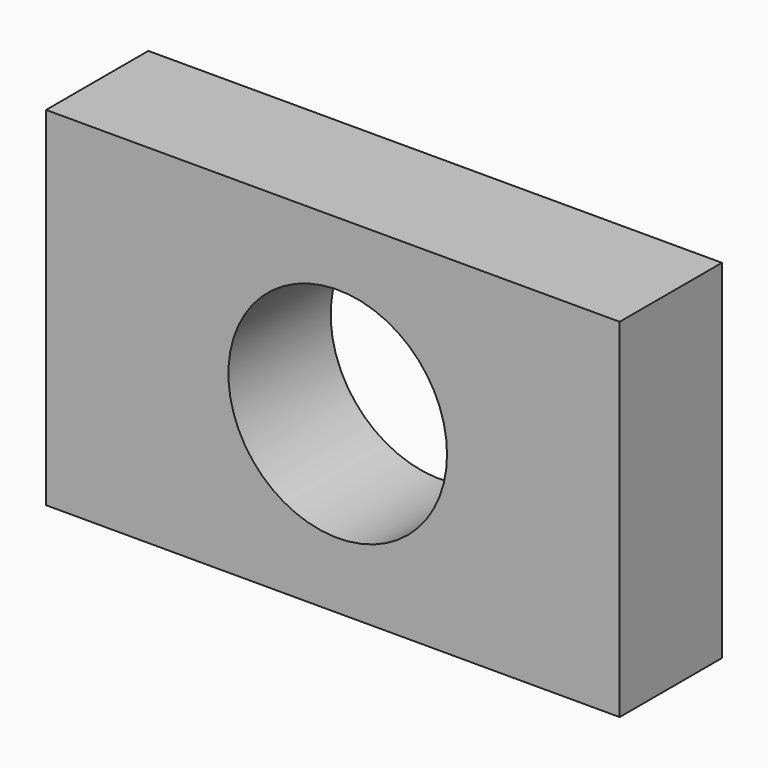
from build123d import *

# Parameters (mm, degrees)
F0_W     = 113.9901466668
F0_H     = 69.1652707756
F0_R     = 21.7240856747
F2_DEPTH = 25.4


# Not quite as in the source:
# - the program builds the solid bodies; features that only make, move or delete a surface that nothing else refers to are left out


with BuildPart() as f2:
    # F0 (on Front) → F2 (new body)
    with BuildSketch(Plane.XZ):
        with Locations((-0.9639766067, -0.2409946173)):
            Rectangle(F0_W, F0_H)
        Circle(F0_R, mode=Mode.SUBTRACT)
    extrude(amount=F2_DEPTH)


solid = f2.part
